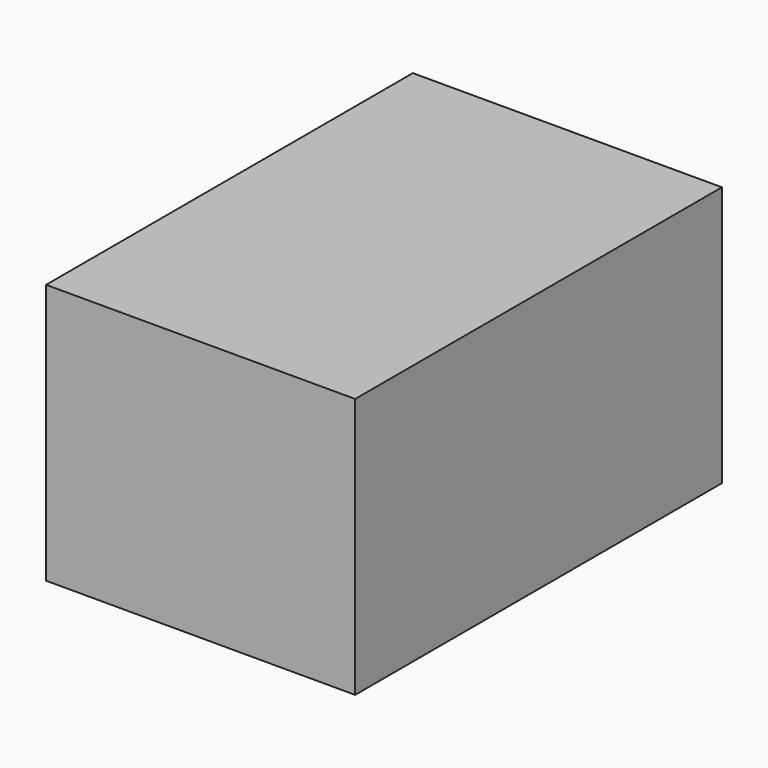
from build123d import *

# Parameters (mm, degrees)
F1_E0_W  = 102.7695015073
F1_E0_H  = 180.848
F2_DEPTH = 121.92


with BuildPart() as f2:
    # F1_E0 (on explicit) → F2 (new body)
    with BuildSketch(Plane(origin=(-144.5072889328, 0, 74.0577951074), x_dir=(0, 0, -1), z_dir=(-1, 0, 0))):
        with Locations((51.3847507536, 90.424)):
            Rectangle(F1_E0_W, F1_E0_H)
    extrude(amount=F2_DEPTH)


solid = f2.part
